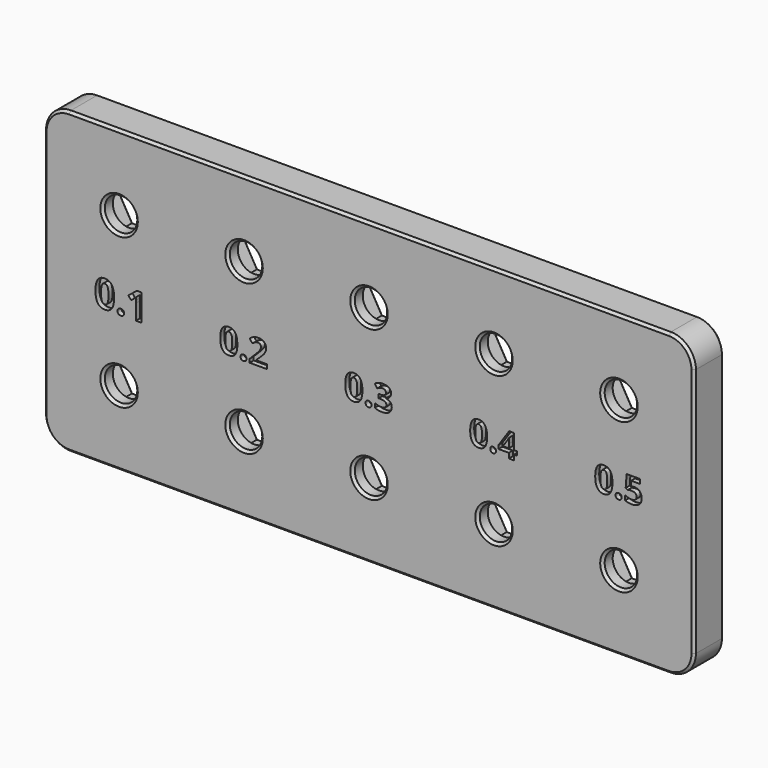
from build123d import *

# Parameters (mm, degrees)
F0_R           = 3.25
F1_DEPTH       = 8
F3_DEPTH       = 5.5
F4_TEXT_SIZE   = 7.4967787279
F4_TEXT_SIZE_2 = 6.8500481644
F4_TEXT_SIZE_3 = 6.8824604796
F4_TEXT_SIZE_4 = 6.7753546475
F4_TEXT_SIZE_5 = 6.9121935414
F5_DEPTH       = 1
F6_SIZE        = 1
F7_SIZE        = 0.5


# Not quite as in the source:
# - Text() gives the source's letters only with a copy of the font that has no kerning and outlines rounded to 1/6400 em; it was checked with that copy


with BuildPart() as f1:
    # F0 (on Front) → F1 (new body)
    with BuildSketch(Plane.XZ):
        with BuildLine():
            ThreePointArc((0, 5), (1.4644660941, 1.4644660941), (5, 0))
            Line((5, 0), (125, 0))
            ThreePointArc((125, 0), (128.5355339059, 1.4644660941), (130, 5))
            Line((130, 5), (130, 55))
            ThreePointArc((130, 55), (128.5355339059, 58.5355339059), (125, 60))
            Line((125, 60), (5, 60))
            ThreePointArc((5, 60), (1.4644660941, 58.5355339059), (0, 55))
            Line((0, 55), (0, 5))
        make_face()
        with Locations((15, 15)):
            Circle(F0_R, mode=Mode.SUBTRACT)
        with Locations((40, 15)):
            Circle(F0_R, mode=Mode.SUBTRACT)
        with Locations((65, 15)):
            Circle(F0_R, mode=Mode.SUBTRACT)
        with Locations((90, 15)):
            Circle(F0_R, mode=Mode.SUBTRACT)
        with Locations((115, 15)):
            Circle(F0_R, mode=Mode.SUBTRACT)
        with Locations((15, 45)):
            Circle(F0_R, mode=Mode.SUBTRACT)
        with Locations((40, 45)):
            Circle(F0_R, mode=Mode.SUBTRACT)
        with Locations((65, 45)):
            Circle(F0_R, mode=Mode.SUBTRACT)
        with Locations((90, 45)):
            Circle(F0_R, mode=Mode.SUBTRACT)
        with Locations((115, 45)):
            Circle(F0_R, mode=Mode.SUBTRACT)
    extrude(amount=F1_DEPTH)

    # F2 (on face) → F3 (cut)
    with BuildSketch(Plane(origin=(0, 0, 0), x_dir=(-1, 0, 0), z_dir=(0, 1, 0))):
        Polygon((-111.9689110868, 39.75), (-108.9378221735, 45), (-111.9689110868, 50.25), (-118.0310889132, 50.25), (-121.0621778265, 45), (-118.0310889132, 39.75), align=None)
        Polygon((-86.9689110868, 50.25), (-93.0310889132, 50.25), (-96.0621778265, 45), (-93.0310889132, 39.75), (-86.9689110868, 39.75), (-83.9378221735, 45), align=None)
        Polygon((-61.9689110868, 50.25), (-68.0310889132, 50.25), (-71.0621778265, 45), (-68.0310889132, 39.75), (-61.9689110868, 39.75), (-58.9378221735, 45), align=None)
        Polygon((-36.9689110868, 50.25), (-43.0310889132, 50.25), (-46.0621778265, 45), (-43.0310889132, 39.75), (-36.9689110868, 39.75), (-33.9378221735, 45), align=None)
        Polygon((-11.9689110868, 50.25), (-18.0310889132, 50.25), (-21.0621778265, 45), (-18.0310889132, 39.75), (-11.9689110868, 39.75), (-8.9378221735, 45), align=None)
        Polygon((-36.9689110868, 20.25), (-43.0310889132, 20.25), (-46.0621778265, 15), (-43.0310889132, 9.75), (-36.9689110868, 9.75), (-33.9378221735, 15), align=None)
        Polygon((-21.0621778265, 15), (-18.0310889132, 9.75), (-11.9689110868, 9.75), (-8.9378221735, 15), (-11.9689110868, 20.25), (-18.0310889132, 20.25), align=None)
        Polygon((-61.9689110868, 20.25), (-68.0310889132, 20.25), (-71.0621778265, 15), (-68.0310889132, 9.75), (-61.9689110868, 9.75), (-58.9378221735, 15), align=None)
        Polygon((-93.0310889132, 20.25), (-96.0621778265, 15), (-93.0310889132, 9.75), (-86.9689110868, 9.75), (-83.9378221735, 15), (-86.9689110868, 20.25), align=None)
        Polygon((-118.0310889132, 9.75), (-111.9689110868, 9.75), (-108.9378221735, 15), (-111.9689110868, 20.25), (-118.0310889132, 20.25), (-121.0621778265, 15), align=None)
    extrude(amount=-F3_DEPTH, mode=Mode.SUBTRACT)

    # F4 (on face) → F5 (cut)
    with BuildSketch(Plane.XZ.offset(8)):
        with Locations((10, 27.5)):
            Text('0.1', F4_TEXT_SIZE, font='Open Sans', font_style=FontStyle.BOLD, text_align=(TextAlign.LEFT, TextAlign.BOTTOM))
        with Locations((35, 27.5)):
            Text('0.2', F4_TEXT_SIZE_2, font='Open Sans', font_style=FontStyle.BOLD, text_align=(TextAlign.LEFT, TextAlign.BOTTOM))
        with Locations((60, 27.5)):
            Text('0.3', F4_TEXT_SIZE_3, font='Open Sans', font_style=FontStyle.BOLD, text_align=(TextAlign.LEFT, TextAlign.BOTTOM))
        with Locations((85, 27.5)):
            Text('0.4', F4_TEXT_SIZE_4, font='Open Sans', font_style=FontStyle.BOLD, text_align=(TextAlign.LEFT, TextAlign.BOTTOM))
        with Locations((110, 27.5)):
            Text('0.5', F4_TEXT_SIZE_5, font='Open Sans', font_style=FontStyle.BOLD, text_align=(TextAlign.LEFT, TextAlign.BOTTOM))
    extrude(amount=-F5_DEPTH, mode=Mode.SUBTRACT)

    # F6
    f6_edges = [f1.edges().sort_by_distance(p)[0] for p in [
        (1.464466, 0, 1.464466),
        (0, 0, 30),
        (65, 0, 0),
        (1.464466, 0, 58.535534),
        (128.535534, 0, 1.464466),
        (65, 0, 60),
        (130, 0, 30),
        (128.535534, 0, 58.535534),
        (15, 0, 20.25),
        (10.453367, 0, 17.625),
        (10.453367, 0, 12.375),
        (15, 0, 9.75),
        (19.546633, 0, 12.375),
        (19.546633, 0, 17.625),
        (35.453367, 0, 12.375),
        (40, 0, 9.75),
        (44.546633, 0, 12.375),
        (44.546633, 0, 17.625),
        (40, 0, 20.25),
        (35.453367, 0, 17.625),
        (60.453367, 0, 12.375),
        (65, 0, 9.75),
        (69.546633, 0, 12.375),
        (69.546633, 0, 17.625),
        (65, 0, 20.25),
        (60.453367, 0, 17.625),
        (90, 0, 20.25),
        (85.453367, 0, 17.625),
        (85.453367, 0, 12.375),
        (90, 0, 9.75),
        (94.546633, 0, 12.375),
        (94.546633, 0, 17.625),
        (119.546633, 0, 12.375),
        (119.546633, 0, 17.625),
        (115, 0, 20.25),
        (110.453367, 0, 17.625),
        (110.453367, 0, 12.375),
        (115, 0, 9.75),
        (10.453367, 0, 42.375),
        (15, 0, 39.75),
        (19.546633, 0, 42.375),
        (19.546633, 0, 47.625),
        (15, 0, 50.25),
        (10.453367, 0, 47.625),
        (35.453367, 0, 42.375),
        (40, 0, 39.75),
        (44.546633, 0, 42.375),
        (44.546633, 0, 47.625),
        (40, 0, 50.25),
        (35.453367, 0, 47.625),
        (60.453367, 0, 42.375),
        (65, 0, 39.75),
        (69.546633, 0, 42.375),
        (69.546633, 0, 47.625),
        (65, 0, 50.25),
        (60.453367, 0, 47.625),
        (85.453367, 0, 47.625),
        (85.453367, 0, 42.375),
        (90, 0, 39.75),
        (94.546633, 0, 42.375),
        (94.546633, 0, 47.625),
        (90, 0, 50.25),
        (119.546633, 0, 42.375),
        (119.546633, 0, 47.625),
        (115, 0, 50.25),
        (110.453367, 0, 47.625),
        (110.453367, 0, 42.375),
        (115, 0, 39.75),
    ]]
    chamfer(f6_edges, length=F6_SIZE)

    # F7
    f7_edges = [f1.edges().sort_by_distance(p)[0] for p in [
        (0, -8, 30),
        (1.464466, -8, 58.535534),
        (11.75, -8, 45),
        (36.75, -8, 45),
        (61.75, -8, 45),
        (86.75, -8, 45),
        (111.75, -8, 45),
        (11.75, -8, 15),
        (36.75, -8, 15),
        (61.75, -8, 15),
        (86.75, -8, 15),
        (111.75, -8, 15),
    ]]
    chamfer(f7_edges, length=F7_SIZE)


solid = f1.part
